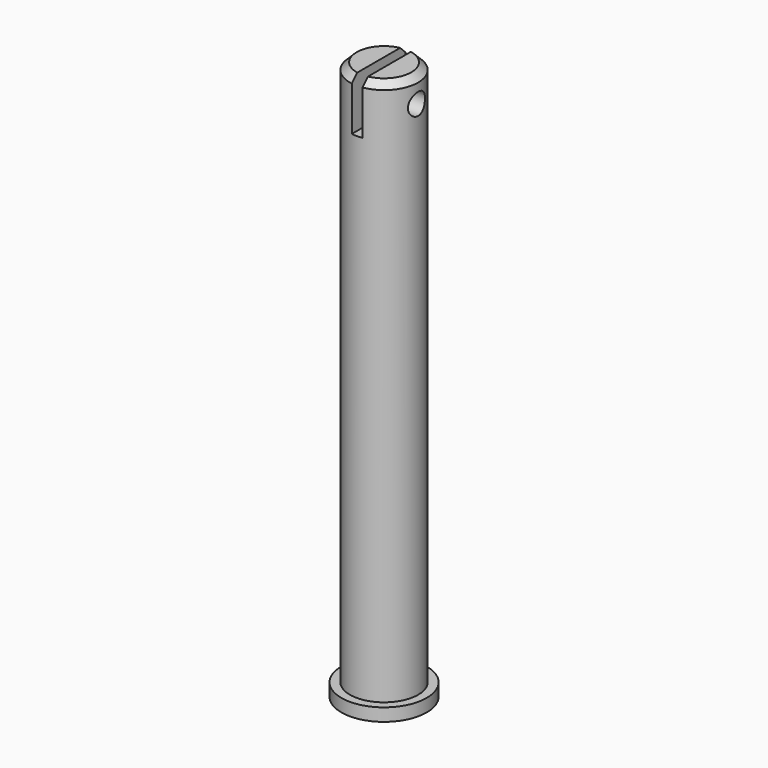
from build123d import *

# Parameters (mm, degrees)
F0_R          = 31.75
F1_DEPTH      = 9.525
F2_R          = 25.4
F3_DEPTH      = 406.4
F5_DEPTH      = 38.1
F6_R          = 7.9375
F7_DEPTH      = 25.4
F7_DEPTH_BACK = 50.8
F8_SIZE       = 5.08


with BuildPart() as f1:
    # F0 (on Top) → F1 (new body)
    with BuildSketch(Plane.XY):
        Circle(F0_R)
    extrude(amount=F1_DEPTH)

    # F2 (on face) → F3 (join)
    with BuildSketch(Plane.XY.offset(9.525)):
        Circle(F2_R)
    extrude(amount=F3_DEPTH)

    # F4 (on face) → F5 (cut)
    with BuildSketch(Plane.XY.offset(415.925)):
        with BuildLine():
            ThreePointArc((3.96875, 25.088025499), (0, 25.4), (-3.96875, 25.088025499))
            Line((-3.96875, 25.088025499), (-3.96875, -25.088025499))
            ThreePointArc((-3.96875, -25.088025499), (0, -25.4), (3.96875, -25.088025499))
            Line((3.96875, -25.088025499), (3.96875, 25.088025499))
        make_face()
    extrude(amount=-F5_DEPTH, mode=Mode.SUBTRACT)

    # F6 (on face) → F7 (cut, two sides)
    with BuildSketch(Plane.YZ.offset(-3.96875)) as f7_sk:
        with Locations((0, 396.875)):
            Circle(F6_R)
    extrude(amount=-F7_DEPTH, mode=Mode.SUBTRACT)
    extrude(f7_sk.sketch, amount=F7_DEPTH_BACK, mode=Mode.SUBTRACT)

    # F8
    f8_edges = [f1.edges().sort_by_distance(p)[0] for p in [
        (-25.4, 0, 415.925),
        (19.312771, -16.497784, 415.925),
        (19.312771, 16.497784, 415.925),
    ]]
    chamfer(f8_edges, length=F8_SIZE)


solid = f1.part
